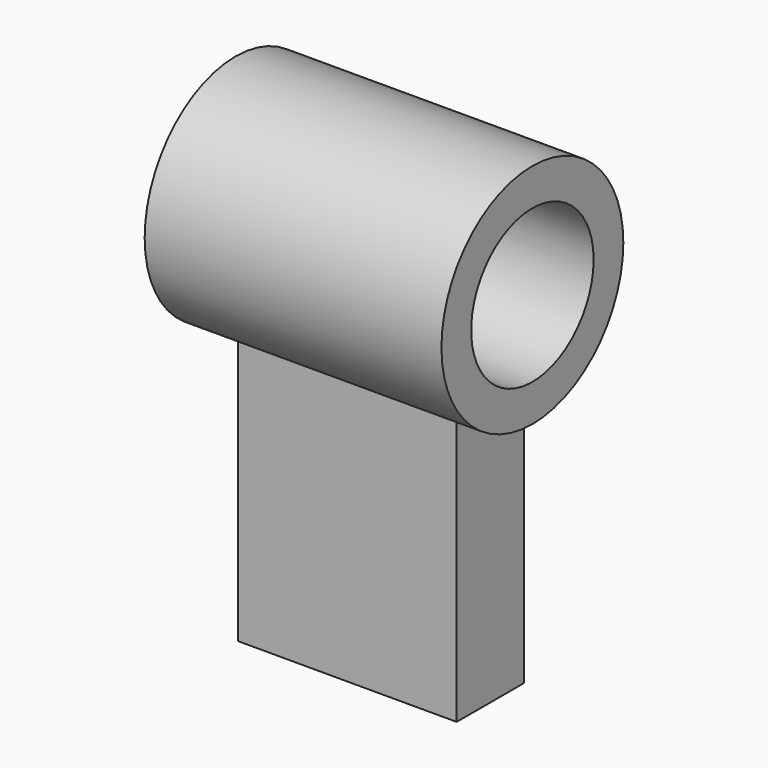
from build123d import *

# Parameters (mm, degrees)
F0_R     = 7.6601757708
F1_DEPTH = 20
F2_W     = 14.7302162368
F2_H     = 5.6654675864
F3_DEPTH = 25
F4_R     = 5.1556537043
F5_DEPTH = 38.2


# Not quite as in the source:
# - a feature of the source that left no trace in its solid (it failed there, or was rolled back) is left out


with BuildPart() as f1:
    # F0 (on Right) → F1 (new body)
    with BuildSketch(Plane.YZ):
        Circle(F0_R)
    extrude(amount=F1_DEPTH)

    # F2 (on Top) → F3 (join)
    with BuildSketch(Plane.XY):
        with Locations((9.9145689746, -0.1416367013)):
            Rectangle(F2_W, F2_H)
    extrude(amount=-F3_DEPTH)

    # F4 (on Right) → F5 (cut)
    with BuildSketch(Plane.YZ):
        Circle(F4_R)
    extrude(amount=F5_DEPTH, mode=Mode.SUBTRACT)


solid = f1.part
